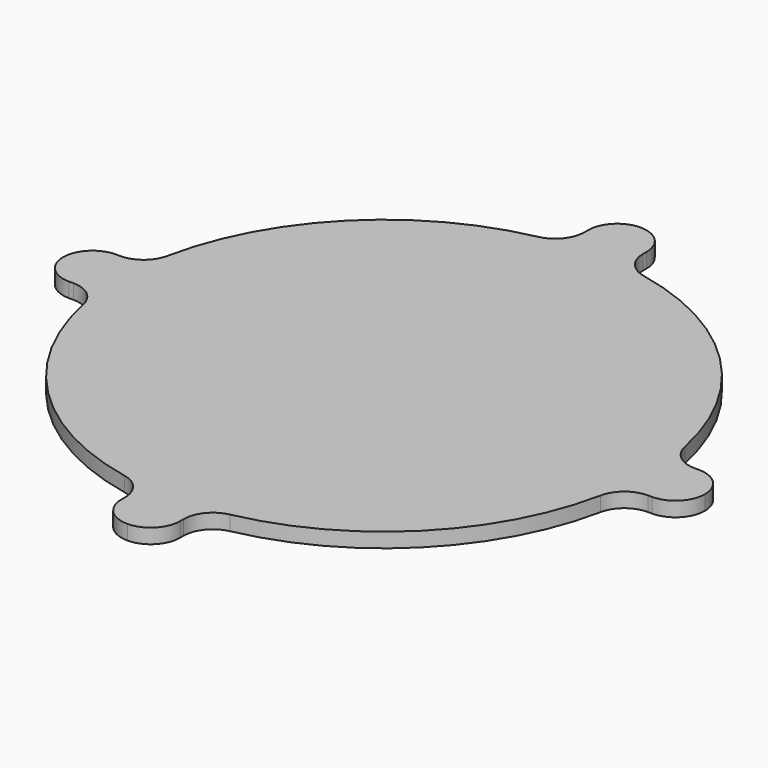
from build123d import *

# Parameters (mm, degrees)
F1_DEPTH = 25.4
F2_R     = 50.79999


# Not quite as in the source:
# - a fillet or chamfer is up to 0.001 mm smaller than in the source, because OpenCascade refuses the exact size


with BuildPart() as f1:
    # F0 (on Top) → F1 (new body)
    with BuildSketch(Plane.XY):
        with BuildLine():
            Line((-50.8, 555.969013028), (-50.8, 454.369013028))
            ThreePointArc((-50.8, 454.369013028), (-323.2892203585, 323.2892203585), (-454.369013028, 50.8))
            Line((-454.369013028, 50.8), (-555.969013028, 50.8))
            Line((-555.969013028, 50.8), (-555.969013028, -50.8))
            Line((-555.969013028, -50.8), (-454.369013028, -50.8))
            ThreePointArc((-454.369013028, -50.8), (-323.2892203585, -323.2892203585), (-50.8, -454.369013028))
            Line((-50.8, -454.369013028), (-50.8, -555.969013028))
            Line((-50.8, -555.969013028), (50.8, -555.969013028))
            Line((50.8, -555.969013028), (50.8, -454.369013028))
            ThreePointArc((50.8, -454.369013028), (323.2892203585, -323.2892203585), (454.369013028, -50.8))
            Line((454.369013028, -50.8), (555.969013028, -50.8))
            Line((555.969013028, -50.8), (555.969013028, 50.8))
            Line((555.969013028, 50.8), (454.369013028, 50.8))
            ThreePointArc((454.369013028, 50.8), (323.2892203585, 323.2892203585), (50.8, 454.369013028))
            Line((50.8, 454.369013028), (50.8, 555.969013028))
            Line((50.8, 555.969013028), (-50.8, 555.969013028))
        make_face()
    extrude(amount=F1_DEPTH)

    # F2 (radius 50.8 in the source; OpenCascade refuses exactly that, so slightly less here)
    f2_edges = [f1.edges().sort_by_distance(p)[0] for p in [
        (50.8, -555.969013, 12.7),
        (-50.8, -555.969013, 12.7),
        (555.969013, -50.8, 12.7),
        (555.969013, 50.8, 12.7),
        (50.8, 555.969013, 12.7),
        (-50.8, 555.969013, 12.7),
        (-555.969013, 50.8, 12.7),
        (-555.969013, -50.8, 12.7),
        (50.8, -454.369013, 12.7),
        (454.369013, -50.8, 12.7),
        (454.369013, 50.8, 12.7),
        (50.8, 454.369013, 12.7),
        (-50.8, 454.369013, 12.7),
        (-454.369013, 50.8, 12.7),
        (-454.369013, -50.8, 12.7),
        (-50.8, -454.369013, 12.7),
    ]]
    fillet(f2_edges, radius=F2_R)


solid = f1.part
